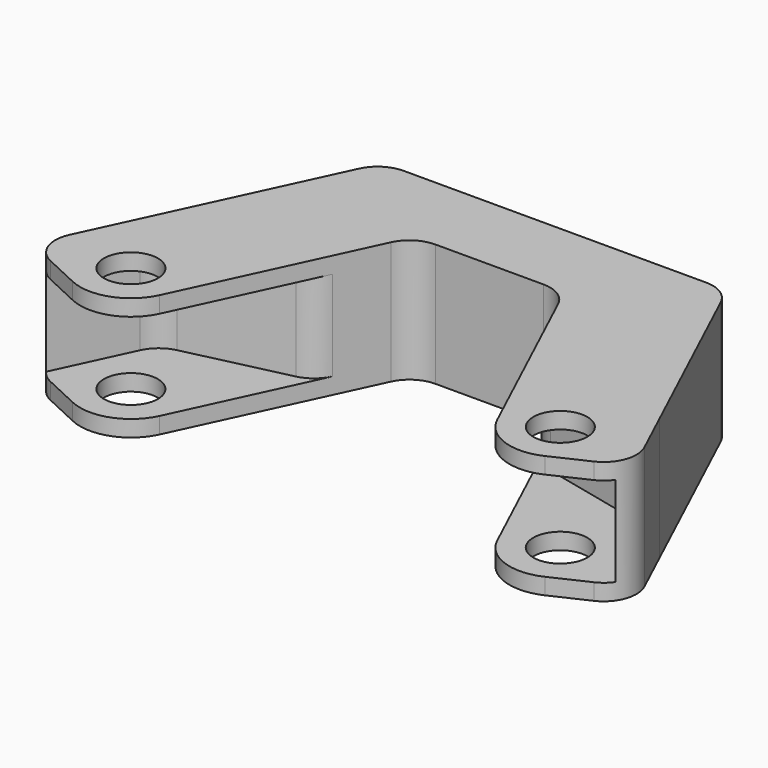
from build123d import *

# Parameters (mm, degrees)
F1_R        = 3.3
F2_DEPTH    = 7.5
F0_R        = 3.3
F3_DEPTH    = 7.501
F5_DEPTH    = 5.5
F6_T1_DEPTH = 15
F6_T3_DEPTH = 11
F6_T5_DEPTH = 11
F6_T7_DEPTH = 35
F6_T9_DEPTH = 27.7414052161


# Not quite as in the source:
# - a fillet or chamfer that OpenCascade refuses, or shapes differently, is made with other operations: its cross-section is extruded or revolved along the edge and cut away or added
# - a feature names something its author has since deleted; it is built from what else it names


with BuildPart() as f2:
    # F1 (on Top) → F2 (new body, symmetric)
    with BuildSketch(Plane.XY):
        with BuildLine():
            Line((-9.150288423, 22), (0, 22))
            Line((0, 22), (9.150288423, 22))
            Line((9.150288423, 22), (20.6308917204, -2.6202332228))
            ThreePointArc((20.6308917204, -2.6202332228), (24.1294751114, -5.8260942489), (28.8702332228, -5.6191082796))
            Line((28.8702332228, -5.6191082796), (36.8457417487, -1.9000675763))
            Line((36.8457417487, -1.9000675763), (32.5785159717, 7.2510276339))
            Line((32.5785159717, 7.2510276339), (21.0378806259, 32))
            Line((21.0378806259, 32), (0, 32))
            Line((0, 32), (-21.0378806259, 32))
            Line((-21.0378806259, 32), (-32.5785159717, 7.2510276339))
            Line((-32.5785159717, 7.2510276339), (-36.8457417487, -1.9000675763))
            Line((-36.8457417487, -1.9000675763), (-28.8702332228, -5.6191082796))
            ThreePointArc((-28.8702332228, -5.6191082796), (-24.1294751114, -5.8260942489), (-20.6308917204, -2.6202332228))
            Line((-20.6308917204, -2.6202332228), (-9.150288423, 22))
        make_face()
        with Locations((-26.25, 0)):
            Circle(F1_R, mode=Mode.SUBTRACT)
        with Locations((26.25, 0)):
            Circle(F1_R, mode=Mode.SUBTRACT)
    extrude(amount=F2_DEPTH, both=True)

    # F0 (on Top) → F3 (cut, through all)
    with BuildSketch(Plane.XY):
        with Locations((26.25, 0)):
            Circle(F0_R)
        with Locations((-26.25, 0)):
            Circle(F0_R)
    extrude(amount=F3_DEPTH, mode=Mode.SUBTRACT)

    # F4 (on Top) → F5 (cut, symmetric)
    with BuildSketch(Plane.XY):
        Polygon((38.163918051, -9.4593089454), (29.7503979029, 8.5835432382), (11.4094827275, 12.8178771483), (24.044580395, -14.2781772408), align=None)
        Polygon((-29.7503979029, 8.5835432382), (-38.163918051, -9.4593089454), (-24.044580395, -14.2781772408), (-11.4094827275, 12.8178771483), align=None)
    extrude(amount=F5_DEPTH, both=True, mode=Mode.SUBTRACT)

    # F6: fillet of radius 4 on 10 edges, made by hand

    # F6_s2 → F6_t1 (join)
    with BuildSketch(Plane.XY.offset(-7.5)):
        with BuildLine():
            ThreePointArc((6.6020073798, 22), (8.7512058132, 21.3735657833), (10.2272385279, 19.690473047))
            Line((10.2272385279, 19.690473047), (9.150288423, 22))
            Line((9.150288423, 22), (6.6020073798, 22))
        make_face()
        with BuildLine():
            ThreePointArc((-10.2272385279, 19.690473047), (-8.7512058132, 21.3735657833), (-6.6020073798, 22))
            Line((-6.6020073798, 22), (-9.150288423, 22))
            Line((-9.150288423, 22), (-10.2272385279, 19.690473047))
        make_face()
    extrude(amount=F6_T1_DEPTH)

    # F6_s4 → F6_t3 (join)
    with BuildSketch(Plane.XY.offset(-5.5)):
        with BuildLine():
            ThreePointArc((27.8494697672, 9.0224070783), (29.466947114, 8.233510665), (30.574896698, 6.8153998661))
            Line((30.574896698, 6.8153998661), (29.7503979029, 8.5835432382))
            Line((29.7503979029, 8.5835432382), (27.8494697672, 9.0224070783))
        make_face()
        with BuildLine():
            ThreePointArc((-30.574896698, 6.8153998661), (-29.466947114, 8.233510665), (-27.8494697672, 9.0224070783))
            Line((-27.8494697672, 9.0224070783), (-29.7503979029, 8.5835432382))
            Line((-29.7503979029, 8.5835432382), (-30.574896698, 6.8153998661))
        make_face()
    extrude(amount=F6_T3_DEPTH)

    # F6_s6 → F6_t5 (cut)
    with BuildSketch(Plane.XY.offset(-5.5)):
        with BuildLine():
            ThreePointArc((12.8514854221, 14.0627574212), (13.9594350061, 12.6446466223), (15.5769123529, 11.855750209))
            Line((15.5769123529, 11.855750209), (13.6759842172, 12.2946140492))
            Line((13.6759842172, 12.2946140492), (12.8514854221, 14.0627574212))
        make_face()
        with BuildLine():
            ThreePointArc((-12.8514854221, 14.0627574212), (-13.9594350061, 12.6446466223), (-15.5769123529, 11.855750209))
            Line((-15.5769123529, 11.855750209), (-13.6759842172, 12.2946140492))
            Line((-13.6759842172, 12.2946140492), (-12.8514854221, 14.0627574212))
        make_face()
    extrude(amount=F6_T5_DEPTH, mode=Mode.SUBTRACT)

    # F6_s8 → F6_t7 (cut)
    with BuildSketch(Plane.XY.offset(-17.5)):
        with BuildLine():
            ThreePointArc((33.2205106006, -3.5905406233), (35.2888080367, -1.3333900484), (35.1552687018, 1.7251635718))
            Line((35.1552687018, 1.7251635718), (36.8457417487, -1.9000675763))
            Line((36.8457417487, -1.9000675763), (33.2205106006, -3.5905406233))
        make_face()
        with BuildLine():
            ThreePointArc((-35.1552687018, 1.7251635718), (-35.2888080367, -1.3333900484), (-33.2205106006, -3.5905406233))
            Line((-33.2205106006, -3.5905406233), (-36.8457417487, -1.9000675763))
            Line((-36.8457417487, -1.9000675763), (-35.1552687018, 1.7251635718))
        make_face()
    extrude(amount=F6_T7_DEPTH, mode=Mode.SUBTRACT)

    # F6_s10 → F6_t9 (cut)
    with BuildSketch(Plane.XY.offset(-13.8707026081)):
        with BuildLine():
            ThreePointArc((18.4895995827, 32), (20.6387980161, 31.3735657833), (22.1148307308, 29.690473047))
            Line((22.1148307308, 29.690473047), (21.0378806259, 32))
            Line((21.0378806259, 32), (18.4895995827, 32))
        make_face()
        with BuildLine():
            ThreePointArc((-22.1148307308, 29.690473047), (-20.6387980161, 31.3735657833), (-18.4895995827, 32))
            Line((-18.4895995827, 32), (-21.0378806259, 32))
            Line((-21.0378806259, 32), (-22.1148307308, 29.690473047))
        make_face()
    extrude(amount=F6_T9_DEPTH, mode=Mode.SUBTRACT)


solid = f2.part
